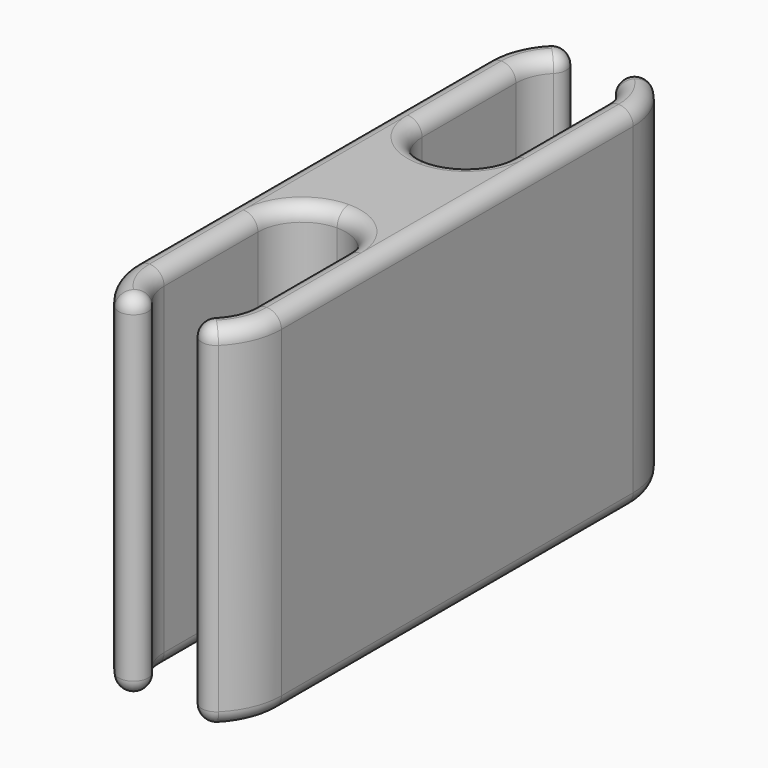
from build123d import *

# Parameters (mm, degrees)
F2_DEPTH = 24
F3_R     = 0.99999


# Not quite as in the source:
# - a fillet or chamfer is up to 0.001 mm smaller than in the source, because OpenCascade refuses the exact size


with BuildPart() as f2:
    # F0 (on Top) → F2 (new body)
    with BuildSketch(Plane.XY):
        with BuildLine():
            ThreePointArc((-2.1213203436, 17.1213203436), (-2.1213203436, 18.5355339059), (-3.5355339059, 18.5355339059))
            ThreePointArc((-3.5355339059, 18.5355339059), (-4.6193976626, 16.9134171618), (-5, 15))
            Line((-5, 15), (-5, 0))
            Line((-5, 0), (-5, -15))
            ThreePointArc((-5, -15), (-4.6193976626, -16.9134171618), (-3.5355339059, -18.5355339059))
            ThreePointArc((-3.5355339059, -18.5355339059), (-2.1213203436, -18.5355339059), (-2.1213203436, -17.1213203436))
            ThreePointArc((-2.1213203436, -17.1213203436), (-2.7716385975, -16.1480502971), (-3, -15))
            Line((-3, -15), (-3, -7))
            ThreePointArc((-3, -7), (-2.1213203436, -4.8786796564), (0, -4))
            ThreePointArc((0, -4), (2.1213203436, -4.8786796564), (3, -7))
            Line((3, -7), (3, -15))
            ThreePointArc((3, -15), (2.7716385975, -16.1480502971), (2.1213203436, -17.1213203436))
            ThreePointArc((2.1213203436, -17.1213203436), (2.1213203436, -18.5355339059), (3.5355339059, -18.5355339059))
            ThreePointArc((3.5355339059, -18.5355339059), (4.6193976626, -16.9134171618), (5, -15))
            Line((5, -15), (5, 0))
            Line((5, 0), (5, 15))
            ThreePointArc((5, 15), (4.6193976626, 16.9134171618), (3.5355339059, 18.5355339059))
            ThreePointArc((3.5355339059, 18.5355339059), (2.1213203436, 18.5355339059), (2.1213203436, 17.1213203436))
            ThreePointArc((2.1213203436, 17.1213203436), (2.7716385975, 16.1480502971), (3, 15))
            Line((3, 15), (3, 7))
            ThreePointArc((3, 7), (2.1213203436, 4.8786796564), (0, 4))
            ThreePointArc((0, 4), (-2.1213203436, 4.8786796564), (-3, 7))
            Line((-3, 7), (-3, 15))
            ThreePointArc((-3, 15), (-2.7716385975, 16.1480502971), (-2.1213203436, 17.1213203436))
        make_face()
    extrude(amount=F2_DEPTH)

    # F3 (radius 1 in the source; OpenCascade refuses exactly that, so slightly less here)
    f3_edges = [f2.edges().sort_by_distance(p)[0] for p in [
        (5, 0, 24),
        (4.619398, 16.913417, 24),
        (2.12132, 18.535534, 24),
        (2.771639, 16.14805, 24),
        (3, 11, 24),
        (0, 4, 24),
        (-3, 11, 24),
        (-2.771639, 16.14805, 24),
        (-2.12132, 18.535534, 24),
        (-4.619398, 16.913417, 24),
        (-5, 0, 24),
        (-4.619398, -16.913417, 24),
        (-2.12132, -18.535534, 24),
        (-2.771639, -16.14805, 24),
        (-3, -11, 24),
        (0, -4, 24),
        (3, -11, 24),
        (2.771639, -16.14805, 24),
        (2.12132, -18.535534, 24),
        (4.619398, -16.913417, 24),
        (5, 0, 0),
        (4.619398, 16.913417, 0),
        (2.12132, 18.535534, 0),
        (2.771639, 16.14805, 0),
        (3, 11, 0),
        (0, 4, 0),
        (-3, 11, 0),
        (-2.771639, 16.14805, 0),
        (-2.12132, 18.535534, 0),
        (-4.619398, 16.913417, 0),
        (-5, 0, 0),
        (-4.619398, -16.913417, 0),
        (-2.12132, -18.535534, 0),
        (-2.771639, -16.14805, 0),
        (-3, -11, 0),
        (0, -4, 0),
        (3, -11, 0),
        (2.771639, -16.14805, 0),
        (2.12132, -18.535534, 0),
        (4.619398, -16.913417, 0),
    ]]
    fillet(f3_edges, radius=F3_R)


solid = f2.part
